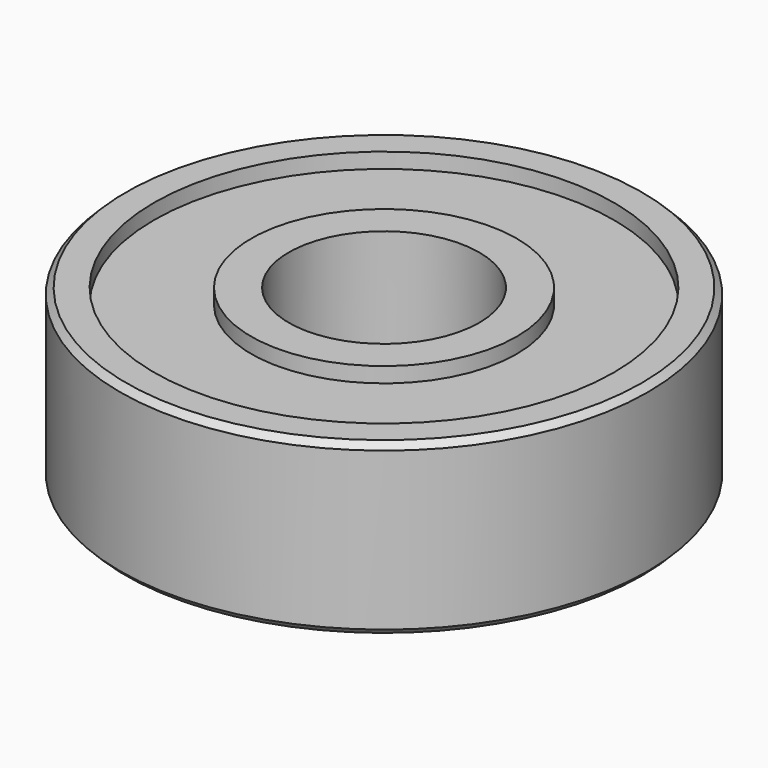
from build123d import *

# Parameters (mm, degrees)
F0_R     = 10.9855
F0_R_2   = 9.5631
F1_DEPTH = 7.0612
F0_R_3   = 5.5245
F0_R_4   = 3.9624
F3_DEPTH = 7.0612
F4_DEPTH = 0.635
F5_DEPTH = 25.4
F6_SIZE  = 0.254


# Not quite as in the source:
# - a pattern or mirror of a feature is missing from the dataset's text; its kind, count and spacing are read off the source's solid


with BuildPart() as f1:
    # F0 (on Top) → F1 (new body)
    with BuildSketch(Plane.XY):
        Circle(F0_R)
        Circle(F0_R_2, mode=Mode.SUBTRACT)
    extrude(amount=F1_DEPTH)

    # F0 (on Top) → F5 (cut)
    with BuildSketch(Plane.XY):
        Circle(F0_R_4)
    extrude(amount=F5_DEPTH, mode=Mode.SUBTRACT)

    # F6
    f6_edges = [f1.edges().sort_by_distance(p)[0] for p in [
        (10.9855, 0, 3.5306),
        (-10.9855, 0, 0),
        (-10.9855, 0, 7.0612),
    ]]
    chamfer(f6_edges, length=F6_SIZE)


with BuildPart() as f1b:
    # F0 (on Top) → F1, piece 2 (new body)
    with BuildSketch(Plane.XY):
        Circle(F0_R_3)
        Circle(F0_R_4, mode=Mode.SUBTRACT)
    extrude(amount=F1_DEPTH)


with BuildPart() as f3:
    # F0 (on Top) → F3 (new body, through all)
    with BuildSketch(Plane.XY):
        Circle(F0_R_2)
        Circle(F0_R_3, mode=Mode.SUBTRACT)
    extrude(amount=F3_DEPTH)

    # F0 (on Top) → F4 (cut)
    with BuildSketch(Plane.XY):
        Circle(F0_R_2)
        Circle(F0_R_3, mode=Mode.SUBTRACT)
    f4 = extrude(amount=F4_DEPTH, mode=Mode.SUBTRACT)

    # F4_copies: F4 across plane
    add(f4.mirror(Plane.XY.offset(3.5306)), mode=Mode.SUBTRACT)


solid = Compound([f1.part, f1b.part, f3.part])
